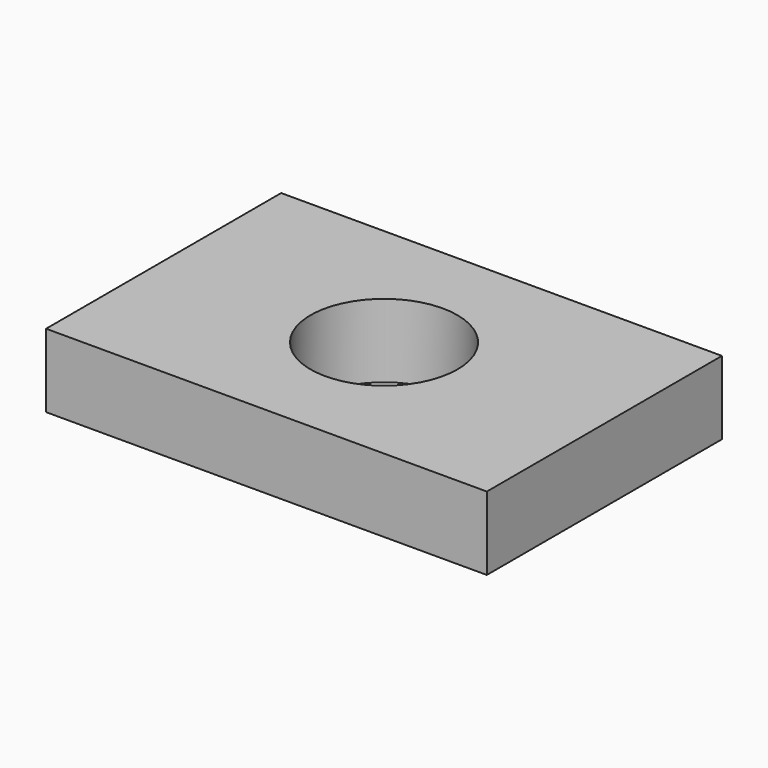
from build123d import *

# Parameters (mm, degrees)
F0_W     = 76.2
F0_H     = 50.8
F0_R     = 12.7
F1_DEPTH = 12.7


# Not quite as in the source:
# - a feature of the source that left no trace in its solid (it failed there, or was rolled back) is left out


with BuildPart() as f1:
    # F0 (on Top) → F1 (new body)
    with BuildSketch(Plane.XY):
        Rectangle(F0_W, F0_H)
        Circle(F0_R, mode=Mode.SUBTRACT)
    extrude(amount=F1_DEPTH)


solid = f1.part
